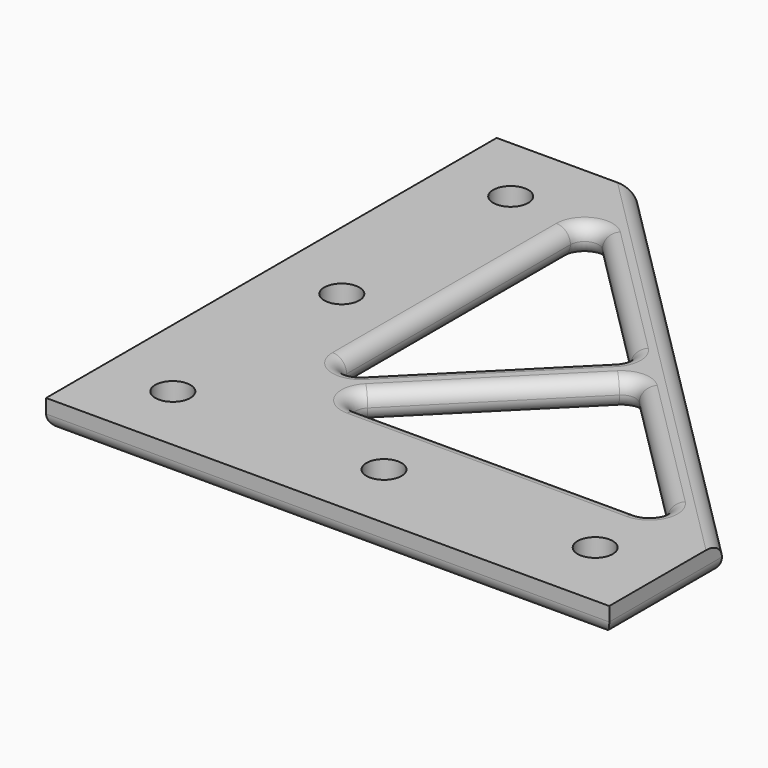
from build123d import *

# Parameters (mm, degrees)
F0_R     = 2.5
F1_DEPTH = 4
F3_DEPTH = 25
F4_R     = 2
F5_R     = 1.99999


# Not quite as in the source:
# - a fillet or chamfer is up to 0.001 mm smaller than in the source, because OpenCascade refuses the exact size


with BuildPart() as f1:
    # F0 (on Top) → F1 (new body)
    with BuildSketch(Plane.XY):
        Polygon((0, 80), (0, 0), (80, 0), (80, 20), (20, 80), align=None)
        with Locations((10, 10)):
            Circle(F0_R, mode=Mode.SUBTRACT)
        with Locations((40, 10)):
            Circle(F0_R, mode=Mode.SUBTRACT)
        with Locations((70, 10)):
            Circle(F0_R, mode=Mode.SUBTRACT)
        with Locations((10, 40)):
            Circle(F0_R, mode=Mode.SUBTRACT)
        with Locations((10, 70)):
            Circle(F0_R, mode=Mode.SUBTRACT)
    extrude(amount=F1_DEPTH)

    # F2 (on face) → F3 (cut)
    with BuildSketch(Plane.XY.offset(4)):
        Polygon((44.6966991411, 48.232233047), (20, 72.9289321881), (20, 23.5355339059), align=None)
        Polygon((23.5355339059, 20), (72.9289321881, 20), (48.232233047, 44.6966991411), align=None)
    extrude(amount=-F3_DEPTH, mode=Mode.SUBTRACT)

    # F4
    f4_edges = [f1.edges().sort_by_distance(p)[0] for p in [
        (80, 10, 0),
        (50, 50, 0),
        (10, 80, 0),
        (0, 40, 0),
        (40, 0, 0),
        (72.928932, 20, 2),
        (48.232233, 44.696699, 2),
        (23.535534, 20, 2),
        (44.696699, 48.232233, 2),
        (20, 23.535534, 2),
        (20, 72.928932, 2),
    ]]
    fillet(f4_edges, radius=F4_R)

    # F5 (radius 2 in the source; OpenCascade refuses exactly that, so slightly less here)
    f5_edges = [f1.edges().sort_by_distance(p)[0] for p in [
        (48.232233, 20, 0),
        (20, 48.232233, 0),
        (50, 50, 4),
        (33.34835, 36.883883, 4),
        (59.580583, 33.34835, 4),
    ]]
    fillet(f5_edges, radius=F5_R)


solid = f1.part
